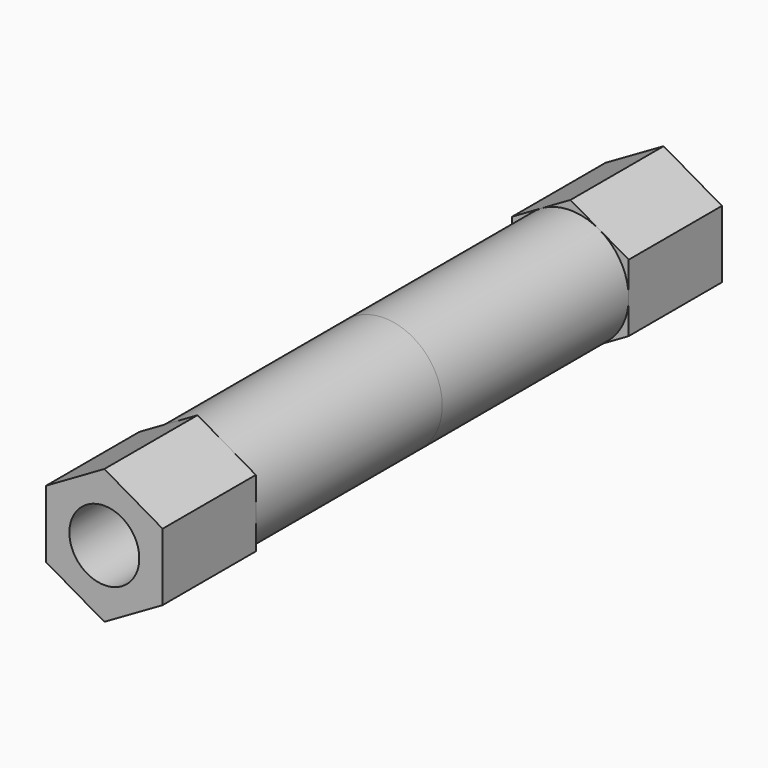
from build123d import *

# Parameters (mm, degrees)
F1_R     = 2.5
F2_DEPTH = 10
F4_DEPTH = 5
F5_D     = 3


# Not quite as in the source:
# - a feature names something its author has since deleted; it is built from what else it names


with BuildPart() as f2:
    # F1 (on Front) → F2 (new body)
    with BuildSketch(Plane.XZ):
        Circle(F1_R)
    extrude(amount=F2_DEPTH)

    # F3 (on face) → F4 (join)
    with BuildSketch(Plane.XZ.offset(10)):
        Polygon((-2.5, 1.443375673), (-2.5, -1.443375673), (0, -2.8867513459), (2.5, -1.443375673), (2.5, 1.443375673), (0, 2.8867513459), align=None)
    extrude(amount=F4_DEPTH)

    # F5 (through all)
    with Locations(Plane(origin=(0, 0, 0), x_dir=(1, 0, 0), z_dir=(0, 1, 0))):
        with Locations((0, 0)):
            Hole(F5_D / 2)

    # F6: F2 across face


with BuildPart() as f2_1:
    add(f2.part)
    add(f2.part.mirror(Plane.XZ))


solid = f2_1.part
